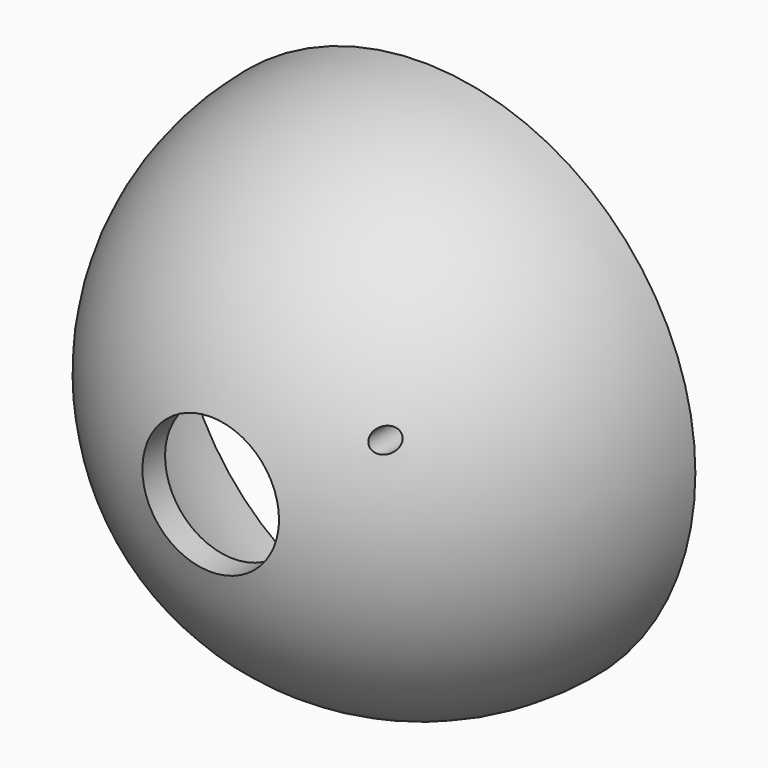
from build123d import *

# Parameters (mm, degrees)
F0_R     = 25.4
F0_R_2   = 1.0439291231
F1_DEPTH = 25.4
F3_T     = -2.54
F4_R     = 6.35
F5_DEPTH = 50.8


# Not quite as in the source:
# - a fillet or chamfer that OpenCascade refuses, or shapes differently, is made with other operations: its cross-section is extruded or revolved along the edge and cut away or added


with BuildPart() as f1:
    # F0 (on Front) → F1 (new body)
    with BuildSketch(Plane.XZ):
        Circle(F0_R)
        with Locations((13.0458941537, 7.0479529987)):
            Circle(F0_R_2, mode=Mode.SUBTRACT)
    extrude(amount=F1_DEPTH)

    # F2: fillet of radius 25.4 on 1 edges, made by hand

    # F2_s1 → F2_t2 (revolve, cut)
    with BuildSketch(Plane.XY):
        with BuildLine():
            ThreePointArc((25.4, 0), (17.9605122421, -17.9605122421), (0, -25.4))
            Line((0, -25.4), (25.4, -25.4))
            Line((25.4, -25.4), (25.4, 0))
        make_face()
    revolve(axis=Axis((0, -25.4, 0), (0, -1, 0)), mode=Mode.SUBTRACT)

    # F3
    f3_openings = [f1.faces().sort_by_distance(p)[0] for p in [
        (-0.022074, 0, -0.011925),
    ]]
    offset(amount=F3_T, openings=f3_openings)

    # F4 (on Front) → F5 (cut)
    with BuildSketch(Plane.XZ):
        Circle(F4_R)
    extrude(amount=F5_DEPTH, mode=Mode.SUBTRACT)


solid = f1.part
